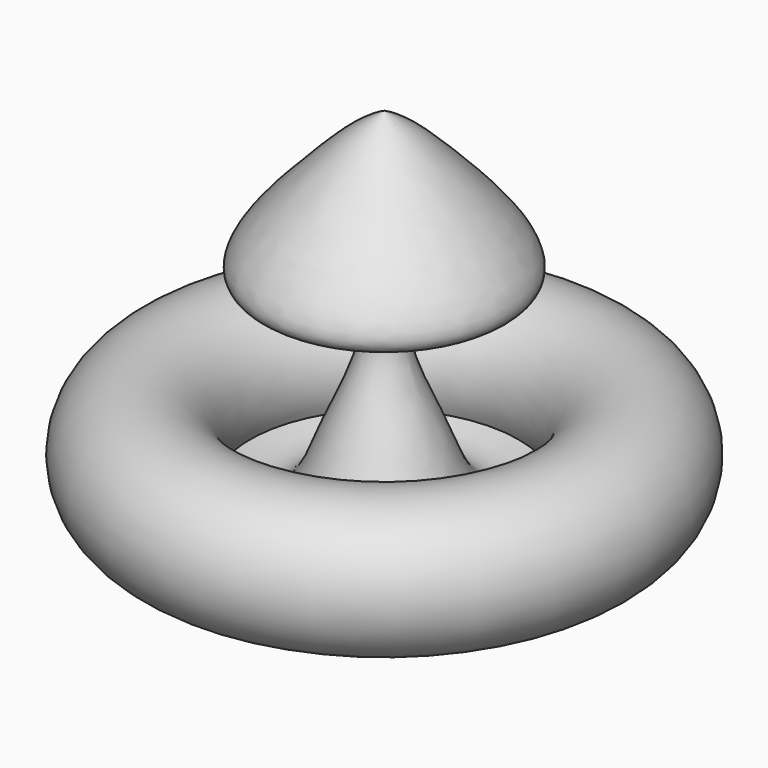
from build123d import *


with BuildPart() as f1:
    # F0 (on Front) → F1 (revolve)
    with BuildSketch(Plane.XZ):
        with BuildLine():
            add(Edge.make_bspline(
                [(0, 77.250353992), (8.6743254896, 72.7689189008), (20.2178919654, 61.5785212547), (59.4759185741, 19.8853143105), (-5.0054218438, 23.86240976), (18.8539341338, -16.5094074623), (24.9545052018, -42.4218556686), (41.7439620239, -37.5708329622), (45.6643509597, -36.0336312152)],
                knots=[0, 0, 0, 0, 0.1251068609, 0.2634519363, 0.3975510306, 0.5305373763, 0.6536601928, 0.6902777855, 0.6902777855, 0.6902777855, 0.6902777855], degree=3))
            Line((0, 77.250353992), (0, -78.1043171883))
            add(Edge.make_bspline(
                [(47.701111507, -39.3533203705), (30.0912414974, -52.2210662947), (5.6716534292, -70.4922042306), (0, -78.1043171883)],
                knots=[0.8664022436, 0.8664022436, 0.8664022436, 0.8664022436, 1, 1, 1, 1], degree=3))
            add(Edge.make_bspline(
                [(45.6643509597, -36.0336312152), (56.1734065387, -31.9129842948), (75.9544012885, -19.0371609293), (57.9781154768, -31.8437887343), (47.701111507, -39.3533203705)],
                knots=[0.6902777855, 0.6902777855, 0.6902777855, 0.6902777855, 0.7884354743, 0.8664022436, 0.8664022436, 0.8664022436, 0.8664022436], degree=3))
        make_face()
        with BuildLine():
            ThreePointArc((47.701111507, -39.3533203705), (86.3756234258, -13.3403170954), (45.6643509597, -36.0336312152))
            add(Edge.make_bspline(
                [(45.6643509597, -36.0336312152), (56.1734065387, -31.9129842948), (75.9544012885, -19.0371609293), (57.9781154768, -31.8437887343), (47.701111507, -39.3533203705)],
                knots=[0.6902777855, 0.6902777855, 0.6902777855, 0.6902777855, 0.7884354743, 0.8664022436, 0.8664022436, 0.8664022436, 0.8664022436], degree=3))
        make_face()
    revolve(axis=Axis((0, 0, -0.4269815981), (0, 0, -1)))


solid = f1.part
